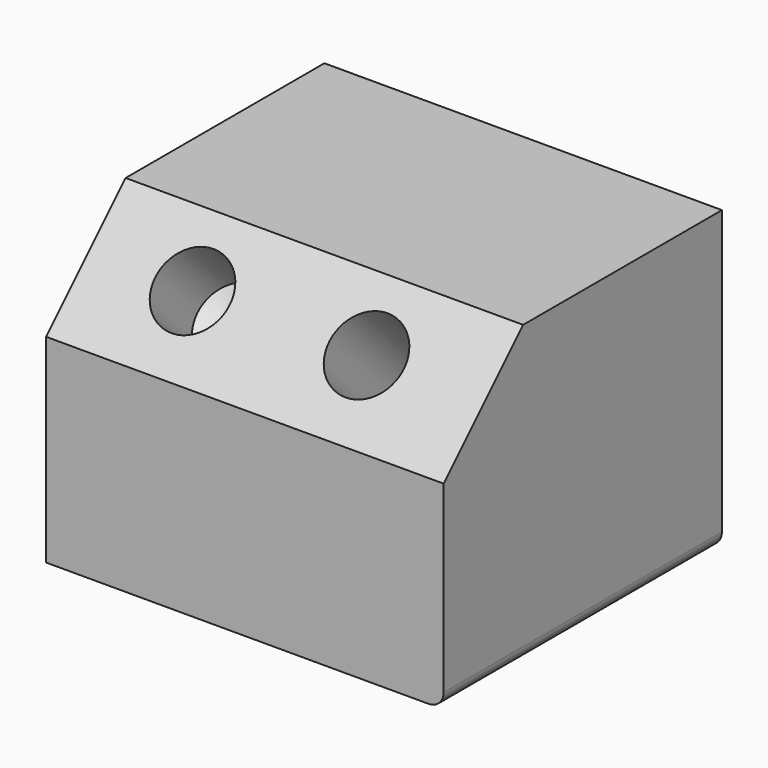
from build123d import *

# Parameters (mm, degrees)
F0_W     = 80
F0_H     = 70
F1_DEPTH = 60
F2_SIZE  = 20
F4_D     = 15
F6_D     = 15
F6_DEPTH = 15
F6_TIP   = 4.5064546427
F7_R     = 3


with BuildPart() as f1:
    # F0 (on Top) → F1 (new body)
    with BuildSketch(Plane.XY):
        with Locations((-40, -35)):
            Rectangle(F0_W, F0_H)
    extrude(amount=F1_DEPTH)

    # F2
    f2_edges = [f1.edges().sort_by_distance(p)[0] for p in [
        (-40, -70, 60),
    ]]
    chamfer(f2_edges, length=F2_SIZE)

    # F4 (through all)
    with Locations(Plane(origin=(0, -55, 55), x_dir=(1, 0, 0), z_dir=(0, -0.7071067812, 0.7071067812))):
        with Locations((-24, -6.2132034356)):
            Hole(F4_D / 2)

    # F6
    with Locations(Plane(origin=(0, -55, 55), x_dir=(1, 0, 0), z_dir=(0, -0.7071067812, 0.7071067812))):
        with Locations((-59.0175294898, -6.2132034356)):
            Hole(F6_D / 2, depth=F6_DEPTH)
            with Locations((0, 0, -(F6_DEPTH + F6_TIP / 2))):  # 118° drill point
                Cone(0, F6_D / 2, F6_TIP, mode=Mode.SUBTRACT)

    # F7
    f7_edges = [f1.edges().sort_by_distance(p)[0] for p in [
        (0, -35, 0),
    ]]
    fillet(f7_edges, radius=F7_R)


solid = f1.part
